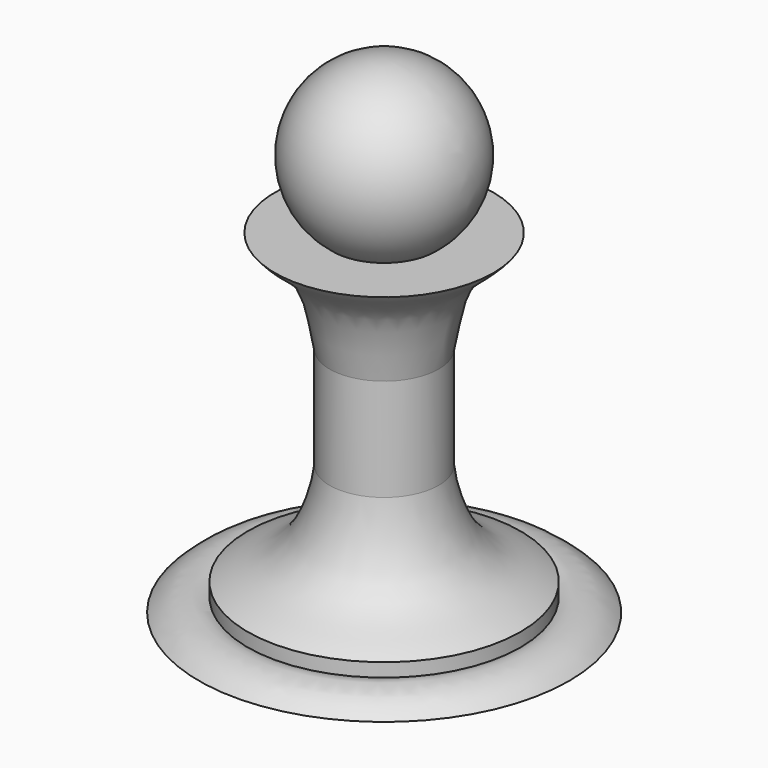
from build123d import *


# Not quite as in the source:
# - a feature names something its author has since deleted; it is built from what else it names


with BuildPart() as f1:
    # F0 (on Front) → F1 (revolve)
    with BuildSketch(Plane.XZ):
        with BuildLine():
            Line((16, -2.4131433771), (7.5, -2.4131433771))
            ThreePointArc((7.5, -2.4131433771), (11.8585412256, 11.5397036981), (0, 20.0868566229))
            Line((0, 20.0868566229), (0, 7.5868566229))
            Line((0, 7.5868566229), (0, -2.4131433771))
            Line((0, -2.4131433771), (0, -17.4131433771))
            Line((0, -17.4131433771), (0, -32.4131433771))
            Line((0, -32.4131433771), (0, -47.4131433771))
            Line((0, -47.4131433771), (0.1347365081, -49.4085997343))
            Line((0.1347365081, -49.4085997343), (0.1347365081, -51.4085997343))
            Line((0.1347365081, -51.4085997343), (27.1347365081, -51.4085997343))
            add(Edge.make_bspline(
                [(20, -49.4085997343), (21.1647466197, -48.7697309267), (24.5158880863, -49.2280358233), (26.0127596557, -50.3029301763), (27.1347365081, -51.4085997343)],
                knots=[0, 0, 0, 0, 0.5171119301, 1, 1, 1, 1], degree=3))
            Line((20, -49.4085997343), (20, -47.4131433771))
            add(Edge.make_bspline(
                [(8, -32.4131433771), (8.1538179197, -34.0022767405), (8.8353543612, -37.329541577), (12.0621827681, -44.6088268089), (17.7756990209, -46.0672005111), (20, -47.4131433771)],
                knots=[0, 0, 0, 0, 0.2858059908, 0.6339622457, 1, 1, 1, 1], degree=3))
            Line((8, -32.4131433771), (8, -17.4131433771))
            add(Edge.make_bspline(
                [(16, -2.4131433771), (14.9209762915, -3.8251770696), (11.0665886907, -6.0967064809), (8.9117025522, -11.4433176222), (8.4714845406, -15.3714061946), (8, -17.4131433771)],
                knots=[0, 0, 0, 0, 0.3360443888, 0.6607253154, 1, 1, 1, 1], degree=3))
        make_face()
    revolve(axis=Axis((0, 0, 13.8368566229), (0, 0, -1)))


solid = f1.part
